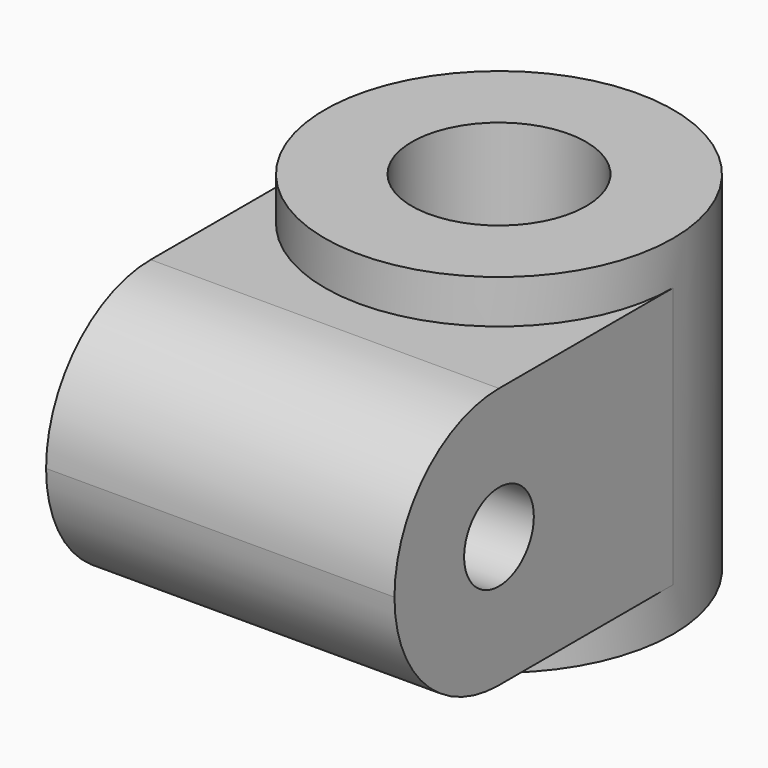
from build123d import *

# Parameters (mm, degrees)
F0_R     = 40
F0_R_2   = 20
F1_DEPTH = 80
F2_W     = 80
F2_H     = 60
F3_DEPTH = 40
F4_DEPTH = 70.001
F5_R     = 29.99999
F6_R     = 10
F7_DEPTH = 80.001


# Not quite as in the source:
# - a fillet or chamfer is up to 0.001 mm smaller than in the source, because OpenCascade refuses the exact size


with BuildPart() as f1:
    # F0 (on Top) → F1 (new body)
    with BuildSketch(Plane.XY):
        Circle(F0_R)
        Circle(F0_R_2, mode=Mode.SUBTRACT)
    extrude(amount=F1_DEPTH)

    # F2 (on Right) → F3 (join, symmetric)
    with BuildSketch(Plane.YZ):
        with Locations((-40, 40)):
            Rectangle(F2_W, F2_H)
    extrude(amount=F3_DEPTH, both=True)

    # F4 (cut, through all): a face of the model
    f4_faces = [f1.faces().sort_by_distance(p)[0] for p in [
        (0, -8.4882636316, 70),
    ]]
    extrude(f4_faces, amount=-F4_DEPTH, mode=Mode.SUBTRACT)

    # F5 (radius 30 in the source; OpenCascade refuses exactly that, so slightly less here)
    f5_edges = [f1.edges().sort_by_distance(p)[0] for p in [
        (0, -80, 70),
        (0, -80, 10),
    ]]
    fillet(f5_edges, radius=F5_R)

    # F6 (on face) → F7 (cut, through all)
    with BuildSketch(Plane.YZ.offset(40)):
        with Locations((-50, 40)):
            Circle(F6_R)
    extrude(amount=-F7_DEPTH, mode=Mode.SUBTRACT)


solid = f1.part
